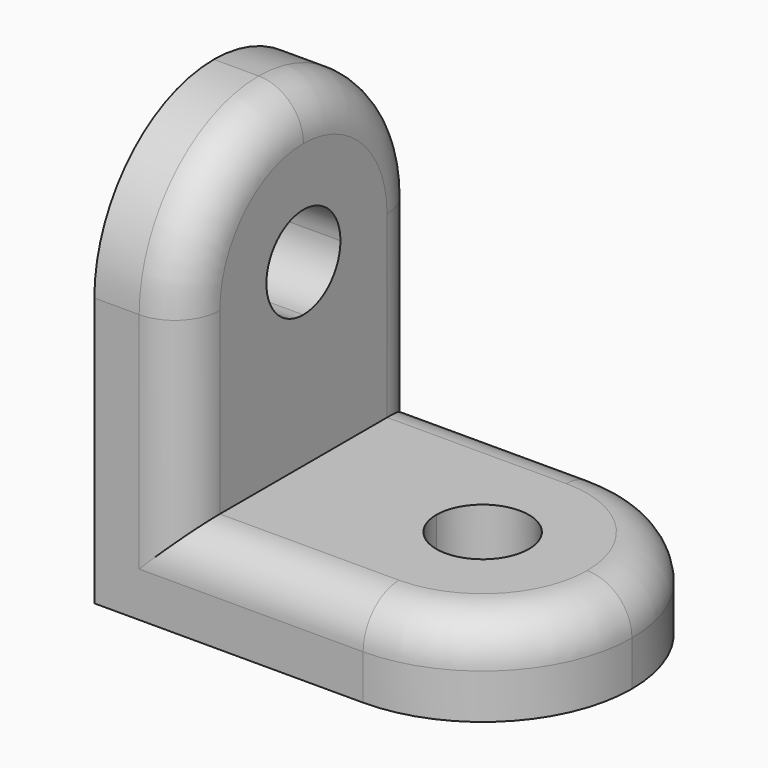
from build123d import *

# Parameters (mm, degrees)
F0_W     = 3
F0_H     = 5
F1_DEPTH = 3
F2_W     = 3
F2_H     = 10
F3_DEPTH = 11
F5_DEPTH = 25
F6_R     = 4.99999
F7_R     = 1.5


# Not quite as in the source:
# - a fillet or chamfer is up to 0.001 mm smaller than in the source, because OpenCascade refuses the exact size


with BuildPart() as f1:
    # F0 (on Top) → F1 (new body)
    with BuildSketch(Plane.XY):
        with Locations((-6.4029270411, -0.9220428518)):
            Rectangle(F0_W, F0_H)
        with Locations((-6.4029270411, -5.9220428518)):
            Rectangle(F0_W, F0_H)
        with BuildLine():
            Line((-4.9029270411, 1.5779571482), (-4.9029270411, -3.4220428518))
            Line((-4.9029270411, -3.4220428518), (-0.4529270411, -3.4220428518))
            ThreePointArc((-0.4529270411, -3.4220428518), (1.0970729589, -1.8720428518), (2.6470729589, -3.4220428518))
            ThreePointArc((2.6470729589, -3.4220428518), (2.1930884698, -4.5180583627), (1.0970729589, -4.9720428518))
            Line((1.0970729589, -4.9720428518), (1.0970729589, -8.4220428518))
            ThreePointArc((1.0970729589, -8.4220428518), (4.6326068649, -6.9575767578), (6.0970729589, -3.4220428518))
            ThreePointArc((6.0970729589, -3.4220428518), (4.6326068649, 0.1134910541), (1.0970729589, 1.5779571482))
            Line((1.0970729589, 1.5779571482), (-4.9029270411, 1.5779571482))
        make_face()
        with BuildLine():
            Line((-0.4529270411, -3.4220428518), (-4.9029270411, -3.4220428518))
            Line((-4.9029270411, -3.4220428518), (-4.9029270411, -8.4220428518))
            Line((-4.9029270411, -8.4220428518), (1.0970729589, -8.4220428518))
            Line((1.0970729589, -8.4220428518), (1.0970729589, -4.9720428518))
            ThreePointArc((1.0970729589, -4.9720428518), (0.0010574481, -4.5180583627), (-0.4529270411, -3.4220428518))
        make_face()
    extrude(amount=F1_DEPTH)

    # F2 (on face) → F3 (join)
    with BuildSketch(Plane.XY.offset(3)):
        with Locations((-6.4029270411, -3.4220428518)):
            Rectangle(F2_W, F2_H)
    extrude(amount=F3_DEPTH)

    # F4 (on face) → F5 (cut)
    with BuildSketch(Plane.YZ.offset(-4.9029270411)):
        with BuildLine():
            ThreePointArc((-1.8720428518, 9), (-4.5180583627, 10.0960155108), (-3.4220428518, 7.45))
            Line((-3.4220428518, 7.45), (-3.4220428518, 9))
            Line((-3.4220428518, 9), (-1.8720428518, 9))
        make_face()
        with BuildLine():
            Line((-3.4220428518, 9), (-3.4220428518, 7.45))
            ThreePointArc((-3.4220428518, 7.45), (-2.326027341, 7.9039844892), (-1.8720428518, 9))
            Line((-1.8720428518, 9), (-3.4220428518, 9))
        make_face()
    extrude(amount=-F5_DEPTH, mode=Mode.SUBTRACT)

    # F6 (radius 5 in the source; OpenCascade refuses exactly that, so slightly less here)
    f6_edges = [f1.edges().sort_by_distance(p)[0] for p in [
        (-6.402927, -8.422043, 14),
        (-6.402927, 1.577957, 14),
    ]]
    fillet(f6_edges, radius=F6_R)

    # F7
    f7_edges = [f1.edges().sort_by_distance(p)[0] for p in [
        (-4.902927, -6.95758, 12.535537),
        (-4.902927, -8.422043, 6.000005),
        (-1.902927, -8.422043, 3),
    ]]
    fillet(f7_edges, radius=F7_R)


solid = f1.part
